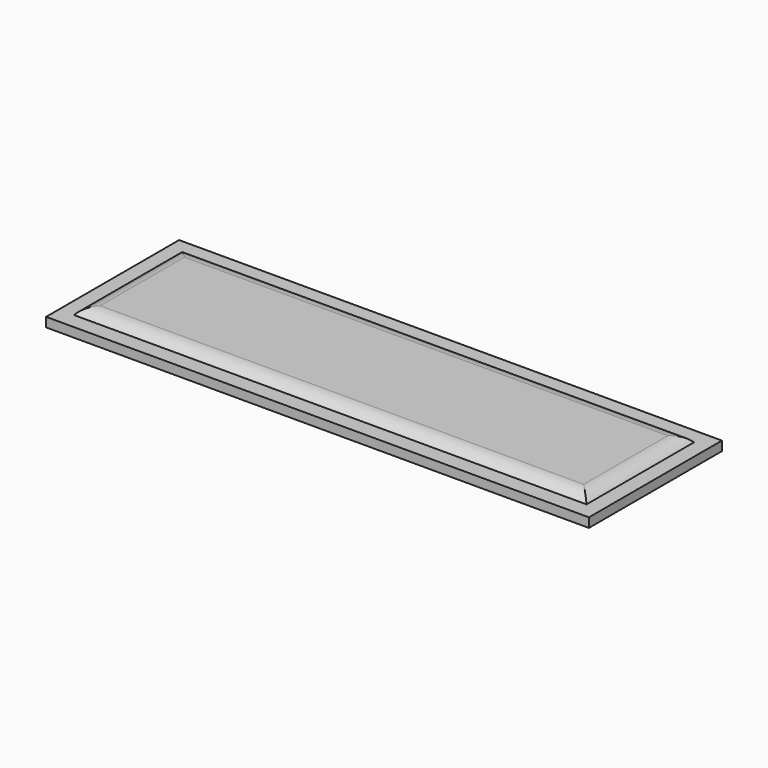
from build123d import *

# Parameters (mm, degrees)
F0_W        = 147.7690637112
F0_H        = 45.2575087547
F1_DEPTH    = 2.54
F2_W        = 139.5183503628
F2_H        = 36.5658290684
F3_DEPTH    = 1.905
F4_T1_DEPTH = 159.3462190077
F4_T3_DEPTH = 56.3936977133


# Not quite as in the source:
# - a fillet or chamfer that OpenCascade refuses, or shapes differently, is made with other operations: its cross-section is extruded or revolved along the edge and cut away or added


with BuildPart() as f1:
    # F0 (on Top) → F1 (new body)
    with BuildSketch(Plane.XY):
        Rectangle(F0_W, F0_H)
    extrude(amount=F1_DEPTH)

    # F2 (on face) → F3 (join)
    with BuildSketch(Plane.XY.offset(2.54)):
        Rectangle(F2_W, F2_H)
    extrude(amount=F3_DEPTH)

    # F4: fillet of radius 5.08 on 4 edges, made by hand

    # F4_s2 → F4_t1 (cut)
    with BuildSketch(Plane.YZ.offset(-79.6731095038)):
        with BuildLine():
            ThreePointArc((-18.2829145342, 2.54), (-16.5170453308, 3.9440501198), (-14.3173408052, 4.445))
            Line((-14.3173408052, 4.445), (-18.2829145342, 4.445))
            Line((-18.2829145342, 4.445), (-18.2829145342, 2.54))
        make_face()
        with BuildLine():
            ThreePointArc((18.2829145342, 2.54), (16.5170453308, 3.9440501198), (14.3173408052, 4.445))
            Line((14.3173408052, 4.445), (18.2829145342, 4.445))
            Line((18.2829145342, 4.445), (18.2829145342, 2.54))
        make_face()
    extrude(amount=F4_T1_DEPTH, mode=Mode.SUBTRACT)

    # F4_s4 → F4_t3 (cut)
    with BuildSketch(Plane.XZ.offset(-28.1968488567)):
        with BuildLine():
            ThreePointArc((-69.7591751814, 2.54), (-67.993305978, 3.9440501198), (-65.7936014524, 4.445))
            Line((-65.7936014524, 4.445), (-69.7591751814, 4.445))
            Line((-69.7591751814, 4.445), (-69.7591751814, 2.54))
        make_face()
        with BuildLine():
            ThreePointArc((69.7591751814, 2.54), (67.993305978, 3.9440501198), (65.7936014524, 4.445))
            Line((65.7936014524, 4.445), (69.7591751814, 4.445))
            Line((69.7591751814, 4.445), (69.7591751814, 2.54))
        make_face()
    extrude(amount=F4_T3_DEPTH, mode=Mode.SUBTRACT)


solid = f1.part
